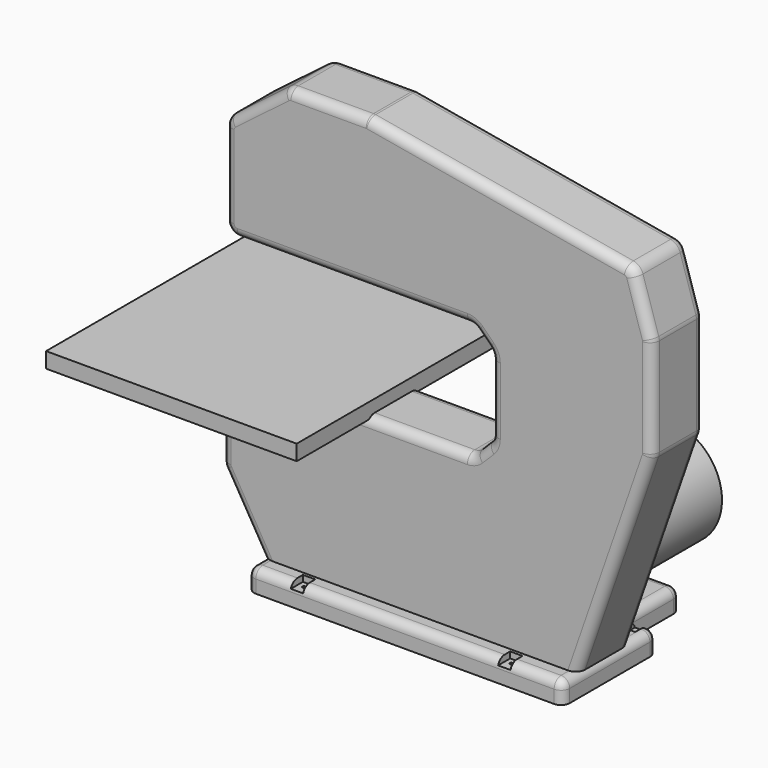
from build123d import *

# Parameters (mm, degrees)
F1_DEPTH       = 44.45
F2_R           = 17.78
F3_R           = 17.78
F4_W           = 25.4
F4_H           = 31.75
F5_DEPTH       = 12.7
F6_R           = 3.175
F7_DEPTH       = 31.751
F10_DEPTH      = 133.35
F11_R          = 25.4
F12_T1_DEPTH   = 201.3434617691
F12_T3_DEPTH   = 107.1700920435
F12_T5_DEPTH   = 536.708406307
F12_T7_DEPTH   = 154.3353423128
F12_T9_DEPTH   = 138.4421511512
F12_T11_DEPTH  = 170.1569830283
F12_T13_DEPTH  = 472.0789755157
F12_T15_DEPTH  = 32.8394877579
F12_T17_DEPTH  = 137.7079510314
F12_T19_DEPTH  = 32.8394877579
F12_T21_DEPTH  = 433.1235738236
F12_T23_DEPTH  = 52.3454572678
F12_T25_DEPTH  = 125.5866942148
F12_T30_DEPTH  = 507.2315122649
F12_T35_DEPTH  = 507.2315122649
F12_T38_ANGLE  = 19.1790080258
F12_T40_ANGLE  = 17.5255683737
F12_T42_ANGLE  = 62.5805109565
F12_T44_ANGLE  = 9.8939206697
F12_T46_ANGLE  = 37.2733041107
F12_T48_ANGLE  = 52.7266958893
F12_T50_ANGLE  = 90
F12_T52_ANGLE  = 45
F12_T54_ANGLE  = 45
F12_T56_ANGLE  = 45
F12_T58_ANGLE  = 45
F12_T60_ANGLE  = 30.0592596661
F12_T62_ANGLE  = 59.9407403339
F12_T64_ANGLE  = 30.5792268725
F12_T68_DEPTH  = 202.9483358745
F12_T71_ANGLE  = 19.1790080258
F12_T73_ANGLE  = 17.5255683737
F12_T75_ANGLE  = 62.5805109565
F12_T77_ANGLE  = 9.8939206697
F12_T79_ANGLE  = 37.2733041107
F12_T81_ANGLE  = 52.7266958893
F12_T83_ANGLE  = 90
F12_T85_ANGLE  = 45
F12_T87_ANGLE  = 45
F12_T89_ANGLE  = 45
F12_T91_ANGLE  = 45
F12_T93_ANGLE  = 30.0592596661
F12_T95_ANGLE  = 59.9407403339
F12_T97_ANGLE  = 30.5792268725
F12_T101_DEPTH = 202.9483358745
F14_W          = 514.35
F14_H          = 514.35
F15_DEPTH      = 31.75
F16_R          = 108.3503204823
F17_DEPTH      = 292.1


# Not quite as in the source:
# - a fillet or chamfer that OpenCascade refuses, or shapes differently, is made with other operations: its cross-section is extruded or revolved along the edge and cut away or added


with BuildPart() as f1:
    # F0 (on Top) → F1 (new body)
    with BuildSketch(Plane.XY):
        Polygon((0, 241.3), (0, 0), (647.7, 0), (647.7, 241.3), (584.2, 241.3), (584.2, 381), (393.7, 381), (393.7, 241.3), align=None)
    extrude(amount=F1_DEPTH)

    # F2
    f2_edges = [f1.edges().sort_by_distance(p)[0] for p in [
        (647.7, 0, 22.225),
        (647.7, 241.3, 22.225),
        (584.2, 241.3, 22.225),
        (584.2, 381, 22.225),
        (393.7, 381, 22.225),
        (393.7, 241.3, 22.225),
        (0, 241.3, 22.225),
        (0, 0, 22.225),
    ]]
    fillet(f2_edges, radius=F2_R)

    # F3
    f3_edges = [f1.edges().sort_by_distance(p)[0] for p in [
        (323.85, 0, 44.45),
    ]]
    fillet(f3_edges, radius=F3_R)

    # F4 (on face) → F5 (cut)
    with BuildSketch(Plane.XY.offset(44.45)):
        with Locations((101.6, 15.875)):
            Rectangle(F4_W, F4_H)
        with Locations((527.05, 15.875)):
            Rectangle(F4_W, F4_H)
        with Locations((615.95, 225.425)):
            Rectangle(F4_W, F4_H)
        with Locations((101.6, 225.425)):
            Rectangle(F4_W, F4_H)
    extrude(amount=-F5_DEPTH, mode=Mode.SUBTRACT)

    # F6 (on face) → F7 (cut, through all)
    with BuildSketch(Plane.XY.offset(31.75)):
        with Locations((527.05, 19.05)):
            Circle(F6_R)
        with Locations((101.6, 19.05)):
            Circle(F6_R)
        with Locations((101.6, 222.25)):
            Circle(F6_R)
        with Locations((615.95, 222.25)):
            Circle(F6_R)
    extrude(amount=-F7_DEPTH, mode=Mode.SUBTRACT)

    # F9 (on offset) → F10 (join)
    with BuildSketch(Plane.XZ.offset(-38.1)):
        Polygon((-82.55, 184.15), (0, 44.45), (647.7, 44.45), (800.1, 482.6), (800.1, 692.15), (762, 812.8), (215.9, 908.05), (50.8, 908.05), (-76.2, 811.395406723), (-76.2, 603.25), (431.8, 603.25), (469.9, 565.15), (469.9, 406.4), (431.8, 368.3), (-18.6645881295, 368.3), (-82.55, 331.3275873661), align=None)
    extrude(amount=-F10_DEPTH)

    # F11
    f11_edges = [f1.edges().sort_by_distance(p)[0] for p in [
        (-82.55, 104.775, 184.15),
        (-82.55, 104.775, 331.327587),
        (-18.664588, 104.775, 368.3),
        (431.8, 104.775, 368.3),
        (469.9, 104.775, 406.4),
        (469.9, 104.775, 565.15),
        (431.8, 104.775, 603.25),
        (-76.2, 104.775, 603.25),
        (-76.2, 104.775, 811.395407),
        (50.8, 104.775, 908.05),
        (215.9, 104.775, 908.05),
        (762, 104.775, 812.8),
        (800.1, 104.775, 692.15),
        (800.1, 104.775, 482.6),
    ]]
    fillet(f11_edges, radius=F11_R)

    # F12: fillet of radius 19.05 on 2 edges, made by hand

    # F12_s2 → F12_t1 (cut)
    with BuildSketch(Plane.XY.offset(486.891302453)):
        with BuildLine():
            ThreePointArc((781.05, 171.45), (794.5203841816, 165.8703841816), (800.1, 152.4))
            Line((800.1, 152.4), (800.1, 171.45))
            Line((800.1, 171.45), (781.05, 171.45))
        make_face()
        with BuildLine():
            ThreePointArc((800.1, 57.15), (794.5203841816, 43.6796158184), (781.05, 38.1))
            Line((781.05, 38.1), (800.1, 38.1))
            Line((800.1, 38.1), (800.1, 57.15))
        make_face()
    extrude(amount=F12_T1_DEPTH, mode=Mode.SUBTRACT)

    # F12_s4 → F12_t3 (cut)
    with BuildSketch(Plane(origin=(-127.3792521948, 0, 403.3676319501), x_dir=(0, 1, 0), z_dir=(-0.3011313679, 0, 0.9535826651))):
        with BuildLine():
            ThreePointArc((171.45, -952.3395666915), (165.8703841816, -965.8099508731), (152.4, -971.3895666915))
            Line((152.4, -971.3895666915), (171.45, -971.3895666915))
            Line((171.45, -971.3895666915), (171.45, -952.3395666915))
        make_face()
        with BuildLine():
            ThreePointArc((57.15, -971.3895666915), (43.6796158184, -965.8099508731), (38.1, -952.3395666915))
            Line((38.1, -952.3395666915), (38.1, -971.3895666915))
            Line((38.1, -971.3895666915), (57.15, -971.3895666915))
        make_face()
    extrude(amount=F12_T3_DEPTH, mode=Mode.SUBTRACT)

    # F12_s6 → F12_t5 (cut)
    with BuildSketch(Plane(origin=(586.7130755264, 0, -102.3336759639), x_dir=(0, 1, 0), z_dir=(-0.985127563, 0, 0.1718245749))):
        with BuildLine():
            ThreePointArc((171.45, -912.5920093418), (165.8703841816, -926.0623935234), (152.4, -931.6420093418))
            Line((152.4, -931.6420093418), (171.45, -931.6420093418))
            Line((171.45, -931.6420093418), (171.45, -912.5920093418))
        make_face()
        with BuildLine():
            ThreePointArc((57.15, -931.6420093418), (43.6796158184, -926.0623935234), (38.1, -912.5920093418))
            Line((38.1, -912.5920093418), (38.1, -931.6420093418))
            Line((38.1, -931.6420093418), (57.15, -931.6420093418))
        make_face()
    extrude(amount=F12_T5_DEPTH, mode=Mode.SUBTRACT)

    # F12_s8 → F12_t7 (cut)
    with BuildSketch(Plane.YZ.offset(59.3661369045)):
        with BuildLine():
            ThreePointArc((171.45, 889), (165.8703841816, 902.4703841816), (152.4, 908.05))
            Line((152.4, 908.05), (171.45, 908.05))
            Line((171.45, 908.05), (171.45, 889))
        make_face()
        with BuildLine():
            ThreePointArc((57.15, 908.05), (43.6796158184, 902.4703841816), (38.1, 889))
            Line((38.1, 889), (38.1, 908.05))
            Line((38.1, 908.05), (57.15, 908.05))
        make_face()
    extrude(amount=F12_T7_DEPTH, mode=Mode.SUBTRACT)

    # F12_s10 → F12_t9 (cut)
    with BuildSketch(Plane(origin=(462.9622613321, 0, 352.341961194), x_dir=(0, 1, 0), z_dir=(-0.7957557434, 0, -0.6056176986))):
        with BuildLine():
            ThreePointArc((171.45, -672.7706236869), (165.8703841816, -686.2410078685), (152.4, -691.8206236869))
            Line((152.4, -691.8206236869), (171.45, -691.8206236869))
            Line((171.45, -691.8206236869), (171.45, -672.7706236869))
        make_face()
        with BuildLine():
            ThreePointArc((57.15, -691.8206236869), (43.6796158184, -686.2410078685), (38.1, -672.7706236869))
            Line((38.1, -672.7706236869), (38.1, -691.8206236869))
            Line((38.1, -691.8206236869), (57.15, -691.8206236869))
        make_face()
    extrude(amount=F12_T9_DEPTH, mode=Mode.SUBTRACT)

    # F12_s12 → F12_t11 (cut)
    with BuildSketch(Plane.XY.offset(628.65)):
        with BuildLine():
            ThreePointArc((-57.15, 171.45), (-70.6203841816, 165.8703841816), (-76.2, 152.4))
            Line((-76.2, 152.4), (-76.2, 171.45))
            Line((-76.2, 171.45), (-57.15, 171.45))
        make_face()
        with BuildLine():
            ThreePointArc((-76.2, 57.15), (-70.6203841816, 43.6796158184), (-57.15, 38.1))
            Line((-57.15, 38.1), (-76.2, 38.1))
            Line((-76.2, 38.1), (-76.2, 57.15))
        make_face()
    extrude(amount=F12_T11_DEPTH, mode=Mode.SUBTRACT)

    # F12_s14 → F12_t13 (cut)
    with BuildSketch(Plane.YZ.offset(-50.8)):
        with BuildLine():
            ThreePointArc((171.45, 622.3), (165.8703841816, 608.8296158184), (152.4, 603.25))
            Line((152.4, 603.25), (171.45, 603.25))
            Line((171.45, 603.25), (171.45, 622.3))
        make_face()
        with BuildLine():
            ThreePointArc((57.15, 603.25), (43.6796158184, 608.8296158184), (38.1, 622.3))
            Line((38.1, 622.3), (38.1, 603.25))
            Line((38.1, 603.25), (57.15, 603.25))
        make_face()
    extrude(amount=F12_T13_DEPTH, mode=Mode.SUBTRACT)

    # F12_s16 → F12_t15 (cut)
    with BuildSketch(Plane(origin=(-78.2855122421, 0, 78.2855122421), x_dir=(0, 1, 0), z_dir=(0.7071067812, 0, -0.7071067812))):
        with BuildLine():
            ThreePointArc((171.45, 750.9408738671), (165.8703841816, 737.4704896855), (152.4, 731.8908738671))
            Line((152.4, 731.8908738671), (171.45, 731.8908738671))
            Line((171.45, 731.8908738671), (171.45, 750.9408738671))
        make_face()
        with BuildLine():
            ThreePointArc((57.15, 731.8908738671), (43.6796158184, 737.4704896855), (38.1, 750.9408738671))
            Line((38.1, 750.9408738671), (38.1, 731.8908738671))
            Line((38.1, 731.8908738671), (57.15, 731.8908738671))
        make_face()
    extrude(amount=F12_T15_DEPTH, mode=Mode.SUBTRACT)

    # F12_s18 → F12_t17 (cut)
    with BuildSketch(Plane.XY.offset(416.9210244843)):
        with BuildLine():
            ThreePointArc((488.95, 171.45), (475.4796158184, 165.8703841816), (469.9, 152.4))
            Line((469.9, 152.4), (469.9, 171.45))
            Line((469.9, 171.45), (488.95, 171.45))
        make_face()
        with BuildLine():
            ThreePointArc((469.9, 57.15), (475.4796158184, 43.6796158184), (488.95, 38.1))
            Line((488.95, 38.1), (469.9, 38.1))
            Line((469.9, 38.1), (469.9, 57.15))
        make_face()
    extrude(amount=F12_T17_DEPTH, mode=Mode.SUBTRACT)

    # F12_s20 → F12_t19 (cut)
    with BuildSketch(Plane(origin=(430.7105122421, 0, 430.7105122421), x_dir=(0, 1, 0), z_dir=(-0.7071067812, 0, -0.7071067812))):
        with BuildLine():
            ThreePointArc((171.45, 63.9512806053), (165.8703841816, 50.4808964237), (152.4, 44.9012806053))
            Line((152.4, 44.9012806053), (171.45, 44.9012806053))
            Line((171.45, 44.9012806053), (171.45, 63.9512806053))
        make_face()
        with BuildLine():
            ThreePointArc((57.15, 44.9012806053), (43.6796158184, 50.4808964237), (38.1, 63.9512806053))
            Line((38.1, 63.9512806053), (38.1, 44.9012806053))
            Line((38.1, 44.9012806053), (57.15, 44.9012806053))
        make_face()
    extrude(amount=F12_T19_DEPTH, mode=Mode.SUBTRACT)

    # F12_s22 → F12_t21 (cut)
    with BuildSketch(Plane.YZ.offset(-11.8445983079)):
        with BuildLine():
            ThreePointArc((171.45, 349.25), (165.8703841816, 362.7203841816), (152.4, 368.3))
            Line((152.4, 368.3), (171.45, 368.3))
            Line((171.45, 368.3), (171.45, 349.25))
        make_face()
        with BuildLine():
            ThreePointArc((57.15, 368.3), (43.6796158184, 362.7203841816), (38.1, 349.25))
            Line((38.1, 349.25), (38.1, 368.3))
            Line((38.1, 368.3), (57.15, 368.3))
        make_face()
    extrude(amount=F12_T21_DEPTH, mode=Mode.SUBTRACT)

    # F12_s24 → F12_t23 (cut)
    with BuildSketch(Plane(origin=(139.7842312721, 0, 80.8973461544), x_dir=(0, 1, 0), z_dir=(-0.8655078025, 0, -0.5008954419))):
        with BuildLine():
            ThreePointArc((171.45, -309.0655307907), (165.8703841816, -322.5359149723), (152.4, -328.1155307907))
            Line((152.4, -328.1155307907), (171.45, -328.1155307907))
            Line((171.45, -328.1155307907), (171.45, -309.0655307907))
        make_face()
        with BuildLine():
            ThreePointArc((57.15, -328.1155307907), (43.6796158184, -322.5359149723), (38.1, -309.0655307907))
            Line((38.1, -309.0655307907), (38.1, -328.1155307907))
            Line((38.1, -328.1155307907), (57.15, -328.1155307907))
        make_face()
    extrude(amount=F12_T23_DEPTH, mode=Mode.SUBTRACT)

    # F12_s26 → F12_t25 (cut)
    with BuildSketch(Plane.XY.offset(191.0937048331)):
        with BuildLine():
            ThreePointArc((-63.5, 171.45), (-76.9703841816, 165.8703841816), (-82.55, 152.4))
            Line((-82.55, 152.4), (-82.55, 171.45))
            Line((-82.55, 171.45), (-63.5, 171.45))
        make_face()
        with BuildLine():
            ThreePointArc((-82.55, 57.15), (-76.9703841816, 43.6796158184), (-63.5, 38.1))
            Line((-63.5, 38.1), (-82.55, 38.1))
            Line((-82.55, 38.1), (-82.55, 57.15))
        make_face()
    extrude(amount=F12_T25_DEPTH, mode=Mode.SUBTRACT)


with BuildPart() as f12_tool28:
    # F12_s29 → F12_t30 (new body)
    with BuildSketch(Plane(origin=(68.0499893856, 0, 195.6437194835), x_dir=(0, 1, 0), z_dir=(0.3285206249, 0, 0.9444967967))):
        with BuildLine():
            ThreePointArc((57.15, -597.1478334479), (43.6796158184, -591.5682176295), (38.1, -578.0978334479))
            Line((38.1, -578.0978334479), (38.1, -597.1478334479))
            Line((38.1, -597.1478334479), (57.15, -597.1478334479))
        make_face()
    extrude(amount=F12_T30_DEPTH)

    split(bisect_by=Plane.XY.offset(44.45), keep=Keep.TOP)


with BuildPart() as f1_1:
    add(f1.part)

    # F12_t27: cut F12_tool28
    add(f12_tool28.part, mode=Mode.SUBTRACT)


with BuildPart() as f12_tool33:
    # F12_s34 → F12_t35 (new body)
    with BuildSketch(Plane(origin=(68.0499893856, 0, 195.6437194835), x_dir=(0, 1, 0), z_dir=(0.3285206249, 0, 0.9444967967))):
        with BuildLine():
            ThreePointArc((171.45, -578.0978334479), (165.8703841816, -591.5682176295), (152.4, -597.1478334479))
            Line((152.4, -597.1478334479), (171.45, -597.1478334479))
            Line((171.45, -597.1478334479), (171.45, -578.0978334479))
        make_face()
    extrude(amount=F12_T35_DEPTH)

    split(bisect_by=Plane.XY.offset(44.45), keep=Keep.TOP)


with BuildPart() as f1_2:
    add(f1_1.part)

    # F12_t32: cut F12_tool33
    add(f12_tool33.part, mode=Mode.SUBTRACT)

    # F12_s37 → F12_t38 (revolve, cut)
    with BuildSketch(Plane(origin=(234.6860027847, 0, 674.7222580061), x_dir=(0, 1, 0), z_dir=(-0.3285206249, 0, -0.9444967967))):
        with BuildLine():
            ThreePointArc((171.45, 578.0978334479), (165.8703841816, 591.5682176295), (152.4, 597.1478334479))
            Line((152.4, 597.1478334479), (171.45, 597.1478334479))
            Line((171.45, 597.1478334479), (171.45, 578.0978334479))
        make_face()
    revolve(axis=Axis((774.7, 171.45, 486.891302453), (0, -1, 0)), revolution_arc=F12_T38_ANGLE, mode=Mode.SUBTRACT)

    # F12_s39 → F12_t40 (revolve, cut)
    with BuildSketch(Plane.XY.offset(688.2347642221)):
        with BuildLine():
            ThreePointArc((781.05, 171.45), (794.5203841816, 165.8703841816), (800.1, 152.4))
            Line((800.1, 152.4), (800.1, 171.45))
            Line((800.1, 171.45), (781.05, 171.45))
        make_face()
    revolve(axis=Axis((774.7, 171.45, 688.2347642221), (0, -1, 0)), revolution_arc=F12_T40_ANGLE, mode=Mode.SUBTRACT)

    # F12_s41 → F12_t42 (revolve, cut)
    with BuildSketch(Plane(origin=(-159.6515286138, 0, 505.5631739436), x_dir=(0, 1, 0), z_dir=(0.3011313679, 0, -0.9535826651))):
        with BuildLine():
            ThreePointArc((171.45, 952.3395666915), (165.8703841816, 965.8099508731), (152.4, 971.3895666915))
            Line((152.4, 971.3895666915), (171.45, 971.3895666915))
            Line((171.45, 971.3895666915), (171.45, 952.3395666915))
        make_face()
    revolve(axis=Axis((742.427723581, 171.45, 790.4303062156), (0, -1, 0)), revolution_arc=F12_T42_ANGLE, mode=Mode.SUBTRACT)

    # F12_s43 → F12_t44 (revolve, cut)
    with BuildSketch(Plane(origin=(57.9868311627, 0, -10.1139821795), x_dir=(0, 1, 0), z_dir=(0.985127563, 0, -0.1718245749))):
        with BuildLine():
            ThreePointArc((171.45, 912.5920093418), (165.8703841816, 926.0623935234), (152.4, 931.6420093418))
            Line((152.4, 931.6420093418), (171.45, 931.6420093418))
            Line((171.45, 931.6420093418), (171.45, 912.5920093418))
        make_face()
    revolve(axis=Axis((213.7014792173, 171.45, 882.65), (0, -1, 0)), revolution_arc=F12_T44_ANGLE, mode=Mode.SUBTRACT)

    # F12_s45 → F12_t46 (revolve, cut)
    with BuildSketch(Plane.YZ.offset(59.3661369045)):
        with BuildLine():
            ThreePointArc((171.45, 889), (165.8703841816, 902.4703841816), (152.4, 908.05))
            Line((152.4, 908.05), (171.45, 908.05))
            Line((171.45, 908.05), (171.45, 889))
        make_face()
    revolve(axis=Axis((59.3661369045, 171.45, 882.65), (0, -1, 0)), revolution_arc=F12_T46_ANGLE, mode=Mode.SUBTRACT)

    # F12_s47 → F12_t48 (revolve, cut)
    with BuildSketch(Plane(origin=(352.7961244276, 0, 268.4989442224), x_dir=(0, 1, 0), z_dir=(0.7957557434, 0, 0.6056176986))):
        with BuildLine():
            ThreePointArc((171.45, 672.7706236869), (165.8703841816, 686.2410078685), (152.4, 691.8206236869))
            Line((152.4, 691.8206236869), (171.45, 691.8206236869))
            Line((171.45, 691.8206236869), (171.45, 672.7706236869))
        make_face()
    revolve(axis=Axis((-50.8, 171.45, 798.8069830283), (0, -1, 0)), revolution_arc=F12_T48_ANGLE, mode=Mode.SUBTRACT)

    # F12_s49 → F12_t50 (revolve, cut)
    with BuildSketch(Plane.XY.offset(628.65)):
        with BuildLine():
            ThreePointArc((-57.15, 171.45), (-70.6203841816, 165.8703841816), (-76.2, 152.4))
            Line((-76.2, 152.4), (-76.2, 171.45))
            Line((-76.2, 171.45), (-57.15, 171.45))
        make_face()
    revolve(axis=Axis((-50.8, 171.45, 628.65), (0, -1, 0)), revolution_arc=F12_T50_ANGLE, mode=Mode.SUBTRACT)

    # F12_s51 → F12_t52 (revolve, cut)
    with BuildSketch(Plane.YZ.offset(421.2789755157)):
        with BuildLine():
            ThreePointArc((171.45, 622.3), (165.8703841816, 608.8296158184), (152.4, 603.25))
            Line((152.4, 603.25), (171.45, 603.25))
            Line((171.45, 603.25), (171.45, 622.3))
        make_face()
    revolve(axis=Axis((421.2789755157, 171.45, 577.85), (0, 1, 0)), revolution_arc=F12_T52_ANGLE, mode=Mode.SUBTRACT)

    # F12_s53 → F12_t54 (revolve, cut)
    with BuildSketch(Plane(origin=(-55.0644877579, 0, 55.0644877579), x_dir=(0, 1, 0), z_dir=(-0.7071067812, 0, 0.7071067812))):
        with BuildLine():
            ThreePointArc((171.45, -750.9408738671), (165.8703841816, -737.4704896855), (152.4, -731.8908738671))
            Line((152.4, -731.8908738671), (171.45, -731.8908738671))
            Line((171.45, -731.8908738671), (171.45, -750.9408738671))
        make_face()
    revolve(axis=Axis((444.5, 171.45, 554.6289755157), (0, 1, 0)), revolution_arc=F12_T54_ANGLE, mode=Mode.SUBTRACT)

    # F12_s55 → F12_t56 (revolve, cut)
    with BuildSketch(Plane.XY.offset(416.9210244843)):
        with BuildLine():
            ThreePointArc((488.95, 171.45), (475.4796158184, 165.8703841816), (469.9, 152.4))
            Line((469.9, 152.4), (469.9, 171.45))
            Line((469.9, 171.45), (488.95, 171.45))
        make_face()
    revolve(axis=Axis((444.5, 171.45, 416.9210244843), (0, 1, 0)), revolution_arc=F12_T56_ANGLE, mode=Mode.SUBTRACT)

    # F12_s57 → F12_t58 (revolve, cut)
    with BuildSketch(Plane(origin=(407.4894877579, 0, 407.4894877579), x_dir=(0, 1, 0), z_dir=(0.7071067812, 0, 0.7071067812))):
        with BuildLine():
            ThreePointArc((171.45, -63.9512806053), (165.8703841816, -50.4808964237), (152.4, -44.9012806053))
            Line((152.4, -44.9012806053), (171.45, -44.9012806053))
            Line((171.45, -44.9012806053), (171.45, -63.9512806053))
        make_face()
    revolve(axis=Axis((421.2789755157, 171.45, 393.7), (0, 1, 0)), revolution_arc=F12_T58_ANGLE, mode=Mode.SUBTRACT)

    # F12_s59 → F12_t60 (revolve, cut)
    with BuildSketch(Plane.YZ.offset(-11.8445983079)):
        with BuildLine():
            ThreePointArc((171.45, 349.25), (165.8703841816, 362.7203841816), (152.4, 368.3))
            Line((152.4, 368.3), (171.45, 368.3))
            Line((171.45, 368.3), (171.45, 349.25))
        make_face()
    revolve(axis=Axis((-11.8445983079, 171.45, 342.9), (0, -1, 0)), revolution_arc=F12_T60_ANGLE, mode=Mode.SUBTRACT)

    # F12_s61 → F12_t62 (revolve, cut)
    with BuildSketch(Plane(origin=(94.47882958, 0, 54.6777452023), x_dir=(0, 1, 0), z_dir=(0.8655078025, 0, 0.5008954419))):
        with BuildLine():
            ThreePointArc((171.45, 309.0655307907), (165.8703841816, 322.5359149723), (152.4, 328.1155307907))
            Line((152.4, 328.1155307907), (171.45, 328.1155307907))
            Line((171.45, 328.1155307907), (171.45, 309.0655307907))
        make_face()
    revolve(axis=Axis((-57.15, 171.45, 316.6803990479), (0, -1, 0)), revolution_arc=F12_T62_ANGLE, mode=Mode.SUBTRACT)

    # F12_s63 → F12_t64 (revolve, cut)
    with BuildSketch(Plane(origin=(-98.4856808304, 0, 166.6680752515), x_dir=(0, 1, 0), z_dir=(0.5087293121, 0, -0.8609265282))):
        with BuildLine():
            ThreePointArc((171.45, 41.663017924), (165.8703841816, 28.1926337424), (152.4, 22.613017924))
            Line((152.4, 22.613017924), (171.45, 22.613017924))
            Line((171.45, 22.613017924), (171.45, 41.663017924))
        make_face()
    revolve(axis=Axis((-57.15, 171.45, 191.0937048331), (0, 1, 0)), revolution_arc=F12_T64_ANGLE, mode=Mode.SUBTRACT)


with BuildPart() as f12_tool66:
    # F12_s67 → F12_t68 (new body)
    with BuildSketch(Plane(origin=(-98.4856808304, 0, 166.6680752515), x_dir=(0, 1, 0), z_dir=(0.5087293121, 0, -0.8609265282))):
        with BuildLine():
            ThreePointArc((171.45, 41.663017924), (165.8703841816, 28.1926337424), (152.4, 22.613017924))
            Line((152.4, 22.613017924), (171.45, 22.613017924))
            Line((171.45, 22.613017924), (171.45, 41.663017924))
        make_face()
    extrude(amount=F12_T68_DEPTH)

    split(bisect_by=Plane.XY.offset(44.45), keep=Keep.TOP)


with BuildPart() as f1_3:
    add(f1_2.part)

    # F12_t65: cut F12_tool66
    add(f12_tool66.part, mode=Mode.SUBTRACT)

    # F12_s70 → F12_t71 (revolve, cut)
    with BuildSketch(Plane(origin=(234.6860027847, 0, 674.7222580061), x_dir=(0, 1, 0), z_dir=(-0.3285206249, 0, -0.9444967967))):
        with BuildLine():
            ThreePointArc((57.15, 597.1478334479), (43.6796158184, 591.5682176295), (38.1, 578.0978334479))
            Line((38.1, 578.0978334479), (38.1, 597.1478334479))
            Line((38.1, 597.1478334479), (57.15, 597.1478334479))
        make_face()
    revolve(axis=Axis((774.7, 38.1, 486.891302453), (0, -1, 0)), revolution_arc=F12_T71_ANGLE, mode=Mode.SUBTRACT)

    # F12_s72 → F12_t73 (revolve, cut)
    with BuildSketch(Plane.XY.offset(688.2347642221)):
        with BuildLine():
            ThreePointArc((800.1, 57.15), (794.5203841816, 43.6796158184), (781.05, 38.1))
            Line((781.05, 38.1), (800.1, 38.1))
            Line((800.1, 38.1), (800.1, 57.15))
        make_face()
    revolve(axis=Axis((774.7, 38.1, 688.2347642221), (0, -1, 0)), revolution_arc=F12_T73_ANGLE, mode=Mode.SUBTRACT)

    # F12_s74 → F12_t75 (revolve, cut)
    with BuildSketch(Plane(origin=(-159.6515286138, 0, 505.5631739436), x_dir=(0, 1, 0), z_dir=(0.3011313679, 0, -0.9535826651))):
        with BuildLine():
            ThreePointArc((57.15, 971.3895666915), (43.6796158184, 965.8099508731), (38.1, 952.3395666915))
            Line((38.1, 952.3395666915), (38.1, 971.3895666915))
            Line((38.1, 971.3895666915), (57.15, 971.3895666915))
        make_face()
    revolve(axis=Axis((742.427723581, 38.1, 790.4303062156), (0, -1, 0)), revolution_arc=F12_T75_ANGLE, mode=Mode.SUBTRACT)

    # F12_s76 → F12_t77 (revolve, cut)
    with BuildSketch(Plane(origin=(57.9868311627, 0, -10.1139821795), x_dir=(0, 1, 0), z_dir=(0.985127563, 0, -0.1718245749))):
        with BuildLine():
            ThreePointArc((57.15, 931.6420093418), (43.6796158184, 926.0623935234), (38.1, 912.5920093418))
            Line((38.1, 912.5920093418), (38.1, 931.6420093418))
            Line((38.1, 931.6420093418), (57.15, 931.6420093418))
        make_face()
    revolve(axis=Axis((213.7014792173, 38.1, 882.65), (0, -1, 0)), revolution_arc=F12_T77_ANGLE, mode=Mode.SUBTRACT)

    # F12_s78 → F12_t79 (revolve, cut)
    with BuildSketch(Plane.YZ.offset(59.3661369045)):
        with BuildLine():
            ThreePointArc((57.15, 908.05), (43.6796158184, 902.4703841816), (38.1, 889))
            Line((38.1, 889), (38.1, 908.05))
            Line((38.1, 908.05), (57.15, 908.05))
        make_face()
    revolve(axis=Axis((59.3661369045, 38.1, 882.65), (0, -1, 0)), revolution_arc=F12_T79_ANGLE, mode=Mode.SUBTRACT)

    # F12_s80 → F12_t81 (revolve, cut)
    with BuildSketch(Plane(origin=(352.7961244276, 0, 268.4989442224), x_dir=(0, 1, 0), z_dir=(0.7957557434, 0, 0.6056176986))):
        with BuildLine():
            ThreePointArc((57.15, 691.8206236869), (43.6796158184, 686.2410078685), (38.1, 672.7706236869))
            Line((38.1, 672.7706236869), (38.1, 691.8206236869))
            Line((38.1, 691.8206236869), (57.15, 691.8206236869))
        make_face()
    revolve(axis=Axis((-50.8, 38.1, 798.8069830283), (0, -1, 0)), revolution_arc=F12_T81_ANGLE, mode=Mode.SUBTRACT)

    # F12_s82 → F12_t83 (revolve, cut)
    with BuildSketch(Plane.XY.offset(628.65)):
        with BuildLine():
            ThreePointArc((-76.2, 57.15), (-70.6203841816, 43.6796158184), (-57.15, 38.1))
            Line((-57.15, 38.1), (-76.2, 38.1))
            Line((-76.2, 38.1), (-76.2, 57.15))
        make_face()
    revolve(axis=Axis((-50.8, 38.1, 628.65), (0, -1, 0)), revolution_arc=F12_T83_ANGLE, mode=Mode.SUBTRACT)

    # F12_s84 → F12_t85 (revolve, cut)
    with BuildSketch(Plane.YZ.offset(421.2789755157)):
        with BuildLine():
            ThreePointArc((57.15, 603.25), (43.6796158184, 608.8296158184), (38.1, 622.3))
            Line((38.1, 622.3), (38.1, 603.25))
            Line((38.1, 603.25), (57.15, 603.25))
        make_face()
    revolve(axis=Axis((421.2789755157, 38.1, 577.85), (0, 1, 0)), revolution_arc=F12_T85_ANGLE, mode=Mode.SUBTRACT)

    # F12_s86 → F12_t87 (revolve, cut)
    with BuildSketch(Plane(origin=(-55.0644877579, 0, 55.0644877579), x_dir=(0, 1, 0), z_dir=(-0.7071067812, 0, 0.7071067812))):
        with BuildLine():
            ThreePointArc((57.15, -731.8908738671), (43.6796158184, -737.4704896855), (38.1, -750.9408738671))
            Line((38.1, -750.9408738671), (38.1, -731.8908738671))
            Line((38.1, -731.8908738671), (57.15, -731.8908738671))
        make_face()
    revolve(axis=Axis((444.5, 38.1, 554.6289755157), (0, 1, 0)), revolution_arc=F12_T87_ANGLE, mode=Mode.SUBTRACT)

    # F12_s88 → F12_t89 (revolve, cut)
    with BuildSketch(Plane.XY.offset(416.9210244843)):
        with BuildLine():
            ThreePointArc((469.9, 57.15), (475.4796158184, 43.6796158184), (488.95, 38.1))
            Line((488.95, 38.1), (469.9, 38.1))
            Line((469.9, 38.1), (469.9, 57.15))
        make_face()
    revolve(axis=Axis((444.5, 38.1, 416.9210244843), (0, 1, 0)), revolution_arc=F12_T89_ANGLE, mode=Mode.SUBTRACT)

    # F12_s90 → F12_t91 (revolve, cut)
    with BuildSketch(Plane(origin=(407.4894877579, 0, 407.4894877579), x_dir=(0, 1, 0), z_dir=(0.7071067812, 0, 0.7071067812))):
        with BuildLine():
            ThreePointArc((57.15, -44.9012806053), (43.6796158184, -50.4808964237), (38.1, -63.9512806053))
            Line((38.1, -63.9512806053), (38.1, -44.9012806053))
            Line((38.1, -44.9012806053), (57.15, -44.9012806053))
        make_face()
    revolve(axis=Axis((421.2789755157, 38.1, 393.7), (0, 1, 0)), revolution_arc=F12_T91_ANGLE, mode=Mode.SUBTRACT)

    # F12_s92 → F12_t93 (revolve, cut)
    with BuildSketch(Plane.YZ.offset(-11.8445983079)):
        with BuildLine():
            ThreePointArc((57.15, 368.3), (43.6796158184, 362.7203841816), (38.1, 349.25))
            Line((38.1, 349.25), (38.1, 368.3))
            Line((38.1, 368.3), (57.15, 368.3))
        make_face()
    revolve(axis=Axis((-11.8445983079, 38.1, 342.9), (0, -1, 0)), revolution_arc=F12_T93_ANGLE, mode=Mode.SUBTRACT)

    # F12_s94 → F12_t95 (revolve, cut)
    with BuildSketch(Plane(origin=(94.47882958, 0, 54.6777452023), x_dir=(0, 1, 0), z_dir=(0.8655078025, 0, 0.5008954419))):
        with BuildLine():
            ThreePointArc((57.15, 328.1155307907), (43.6796158184, 322.5359149723), (38.1, 309.0655307907))
            Line((38.1, 309.0655307907), (38.1, 328.1155307907))
            Line((38.1, 328.1155307907), (57.15, 328.1155307907))
        make_face()
    revolve(axis=Axis((-57.15, 38.1, 316.6803990479), (0, -1, 0)), revolution_arc=F12_T95_ANGLE, mode=Mode.SUBTRACT)

    # F12_s96 → F12_t97 (revolve, cut)
    with BuildSketch(Plane(origin=(-98.4856808304, 0, 166.6680752515), x_dir=(0, 1, 0), z_dir=(0.5087293121, 0, -0.8609265282))):
        with BuildLine():
            ThreePointArc((57.15, 22.613017924), (43.6796158184, 28.1926337424), (38.1, 41.663017924))
            Line((38.1, 41.663017924), (38.1, 22.613017924))
            Line((38.1, 22.613017924), (57.15, 22.613017924))
        make_face()
    revolve(axis=Axis((-57.15, 38.1, 191.0937048331), (0, 1, 0)), revolution_arc=F12_T97_ANGLE, mode=Mode.SUBTRACT)


with BuildPart() as f12_tool99:
    # F12_s100 → F12_t101 (new body)
    with BuildSketch(Plane(origin=(-98.4856808304, 0, 166.6680752515), x_dir=(0, 1, 0), z_dir=(0.5087293121, 0, -0.8609265282))):
        with BuildLine():
            ThreePointArc((57.15, 22.613017924), (43.6796158184, 28.1926337424), (38.1, 41.663017924))
            Line((38.1, 41.663017924), (38.1, 22.613017924))
            Line((38.1, 22.613017924), (57.15, 22.613017924))
        make_face()
    extrude(amount=F12_T101_DEPTH)

    split(bisect_by=Plane.XY.offset(44.45), keep=Keep.TOP)


with BuildPart() as f1_4:
    add(f1_3.part)

    # F12_t98: cut F12_tool99
    add(f12_tool99.part, mode=Mode.SUBTRACT)

    # F14 (on offset) → F15 (join)
    with BuildSketch(Plane.XY.offset(393.7)):
        with Locations((-41.275, 114.3)):
            Rectangle(F14_W, F14_H)
    extrude(amount=-F15_DEPTH)

    # F16 (on face) → F17 (join)
    with BuildSketch(Plane(origin=(0, 171.45, 0), x_dir=(-1, 0, 0), z_dir=(0, 1, 0))):
        with Locations((-495.3, 171.45)):
            Circle(F16_R)
    extrude(amount=F17_DEPTH)


solid = f1_4.part
